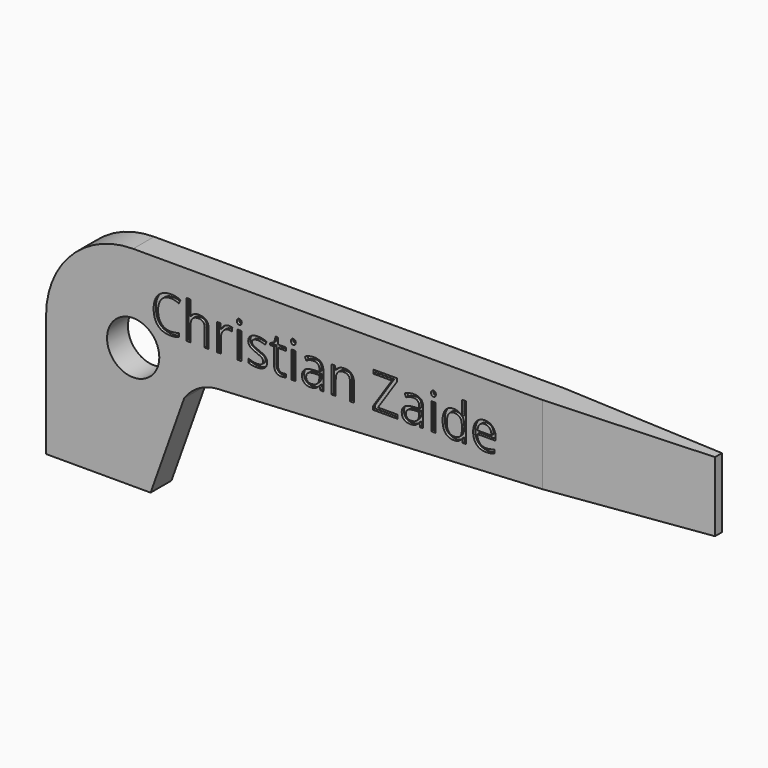
from build123d import *

# Parameters (mm, degrees)
F1_DEPTH     = 2.38125
F2_R         = 2.38125
F3_DEPTH     = 2.38225
F5_DEPTH     = 19.051
F6_TEXT_SIZE = 4.5455562267
F7_DEPTH     = 0.254


# Not quite as in the source:
# - Text() gives the source's letters only with a copy of the font that has no kerning and outlines rounded to 1/6400 em; it was checked with that copy


with BuildPart() as f1:
    # F0 (on Front) → F1 (new body)
    with BuildSketch(Plane.XZ):
        with BuildLine():
            Line((60.325, 19.05), (7.9375, 19.05))
            ThreePointArc((7.9375, 19.05), (2.3248399243, 16.7251600757), (0, 11.1125))
            Line((0, 11.1125), (0, 0))
            Line((0, 0), (9.525, 0))
            Line((9.525, 0), (12.5801754221, 8.5624889973))
            ThreePointArc((12.5801754221, 8.5624889973), (13.9153405853, 9.8011898732), (15.6631963617, 10.3130942181))
            Line((15.6631963617, 10.3130942181), (60.325, 12.7))
            Line((60.325, 12.7), (60.325, 19.05))
        make_face()
    extrude(amount=F1_DEPTH)

    # F2 (on face) → F3 (cut, through all)
    with BuildSketch(Plane.XZ.offset(2.38125)):
        with Locations((7.9375, 11.1125)):
            Circle(F2_R)
    extrude(amount=-F3_DEPTH, mode=Mode.SUBTRACT)

    # F4 (on face) → F5 (cut, through all)
    with BuildSketch(Plane.XY.offset(19.05)):
        Polygon((60.325, 0), (45.24375, 0), (60.325, -0.79375), align=None)
        Polygon((60.325, -2.38125), (60.325, -1.5875), (45.24375, -2.38125), align=None)
    extrude(amount=-F5_DEPTH, mode=Mode.SUBTRACT)

    # F6 (on face) → F7 (cut)
    with BuildSketch(Plane.XZ.offset(2.38125)):
        with Locations((9.525, 13.2371995168)):
            Text('Christian Zaide', F6_TEXT_SIZE, font='Open Sans', text_align=(TextAlign.LEFT, TextAlign.BOTTOM))
    extrude(amount=-F7_DEPTH, mode=Mode.SUBTRACT)


solid = f1.part
